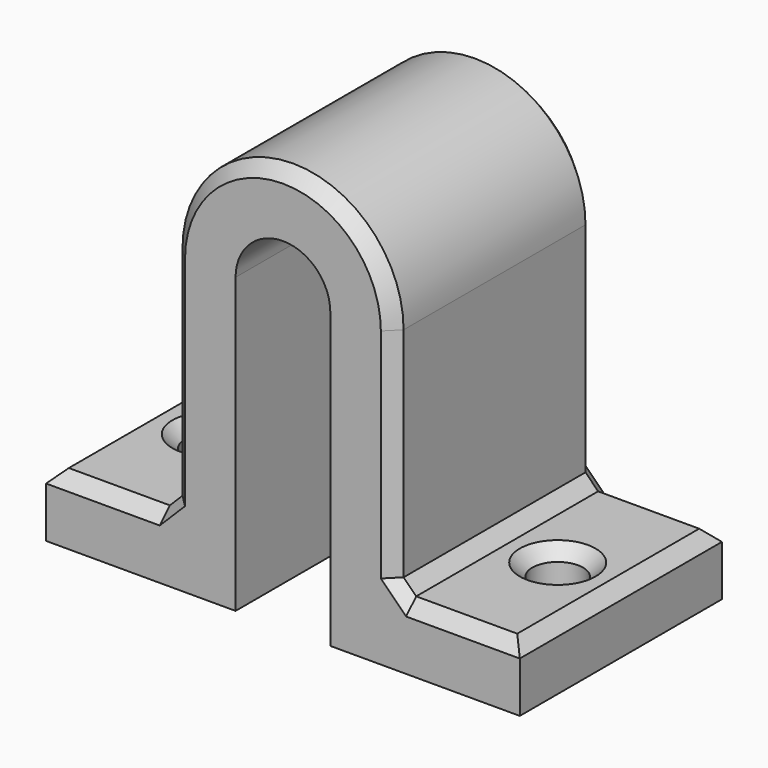
from build123d import *

# Parameters (mm, degrees)
F1_DEPTH      = 10
F1_DEPTH_BACK = 10
F2_R          = 2
F3_DEPTH      = 25
F4_SIZE       = 1


with BuildPart() as f1:
    # F0 (on Front) → F1 (new body, two sides)
    with BuildSketch(Plane.XZ) as f1_sk:
        with BuildLine():
            Line((3.75, 23.25), (3.75, 0))
            Line((3.75, 0), (18.75, 0))
            Line((18.75, 0), (18.75, 5))
            Line((18.75, 5), (8.75, 5))
            Line((8.75, 5), (8.75, 23.25))
            ThreePointArc((8.75, 23.25), (0, 32), (-8.75, 23.25))
            Line((-8.75, 23.25), (-8.75, 5))
            Line((-8.75, 5), (-18.75, 5))
            Line((-18.75, 5), (-18.75, 0))
            Line((-18.75, 0), (-3.75, 0))
            Line((-3.75, 0), (-3.75, 23.25))
            ThreePointArc((-3.75, 23.25), (0, 27), (3.75, 23.25))
        make_face()
    extrude(amount=-F1_DEPTH)
    extrude(f1_sk.sketch, amount=F1_DEPTH_BACK)

    # F2 (on face) → F3 (cut)
    with BuildSketch(Plane.XY.offset(5)):
        with Locations((-13.75, 0)):
            Circle(F2_R)
        with Locations((13.75, 0)):
            Circle(F2_R)
    extrude(amount=-F3_DEPTH, mode=Mode.SUBTRACT)

    # F4
    f4_edges = [f1.edges().sort_by_distance(p)[0] for p in [
        (11.75, 0, 5),
        (-15.75, 0, 5),
        (13.75, -10, 5),
        (18.75, 0, 5),
        (13.75, 10, 5),
        (8.75, 0, 5),
        (-8.75, 0, 5),
        (-13.75, 10, 5),
        (-13.75, -10, 5),
        (-18.75, 0, 5),
        (8.75, 10, 14.125),
        (0, 10, 32),
        (-8.75, 10, 14.125),
        (8.75, -10, 14.125),
        (0, -10, 32),
        (-8.75, -10, 14.125),
    ]]
    chamfer(f4_edges, length=F4_SIZE)


solid = f1.part
